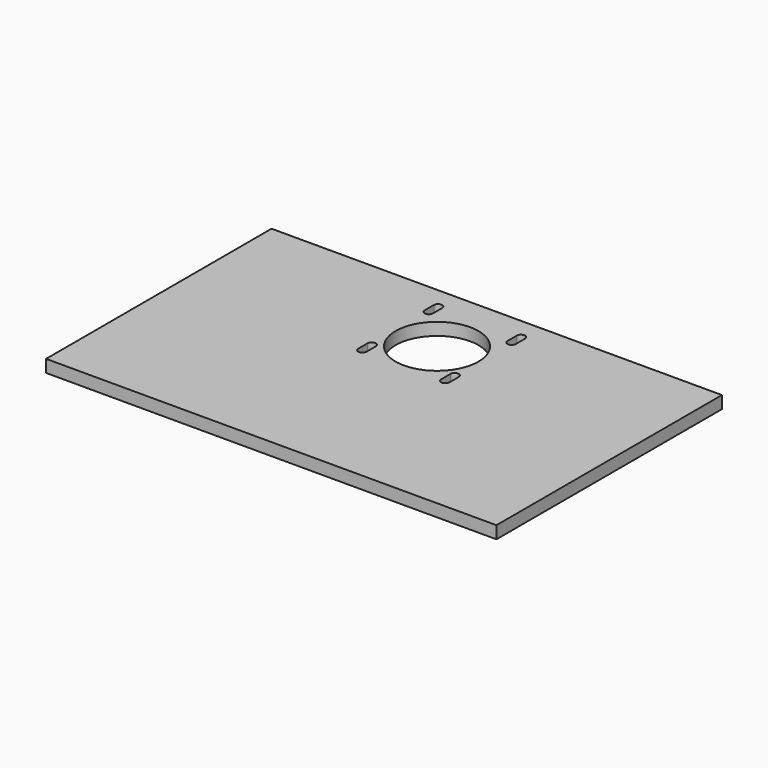
from build123d import *

# Parameters (mm, degrees)
F0_W     = 344.9914
F0_H     = 215.9
F0_R     = 31.75
F1_DEPTH = 9.525


# Not quite as in the source:
# - a length typed as a fraction of an inch, garbled in the dataset ("3 / 203.2 mm" for 3/8 in), is restored


with BuildPart() as f1:
    # F0 (on Top) → F1 (new body)
    with BuildSketch(Plane.XY):
        with Locations((0.0043, -50.8)):
            Rectangle(F0_W, F0_H)
        with BuildLine():
            ThreePointArc((-34.9247077073, -22.903081011), (-31.7715410013, -19.685073074), (-28.575, -22.86))
            Line((-28.575, -22.86), (-28.575, -31.75))
            ThreePointArc((-28.575, -31.75), (-31.7500524496, -34.9249999996), (-34.9249999983, -31.7498951008))
            Line((-34.9249999983, -31.7498951008), (-34.9247077073, -22.903081011))
        make_face(mode=Mode.SUBTRACT)
        Circle(F0_R, mode=Mode.SUBTRACT)
        with BuildLine():
            Line((-28.575, 40.64), (-28.575, 31.75))
            ThreePointArc((-28.575, 31.75), (-31.7500524496, 28.5750000004), (-34.9249999983, 31.7501048992))
            Line((-34.9249999983, 31.7501048992), (-34.9247077073, 40.596918989))
            ThreePointArc((-34.9247077073, 40.596918989), (-31.7715410013, 43.814926926), (-28.575, 40.64))
        make_face(mode=Mode.SUBTRACT)
        with BuildLine():
            ThreePointArc((28.5752922927, -22.903081011), (31.7284589987, -19.685073074), (34.925, -22.86))
            Line((34.925, -22.86), (34.925, -31.75))
            ThreePointArc((34.925, -31.75), (31.7499475504, -34.9249999996), (28.5750000017, -31.7498951008))
            Line((28.5750000017, -31.7498951008), (28.5752922927, -22.903081011))
        make_face(mode=Mode.SUBTRACT)
        with BuildLine():
            ThreePointArc((28.5752922927, 40.596918989), (31.7284589987, 43.814926926), (34.925, 40.64))
            Line((34.925, 40.64), (34.925, 31.75))
            ThreePointArc((34.925, 31.75), (31.7499475504, 28.5750000004), (28.5750000017, 31.7501048992))
            Line((28.5750000017, 31.7501048992), (28.5752922927, 40.596918989))
        make_face(mode=Mode.SUBTRACT)
    extrude(amount=F1_DEPTH)


solid = f1.part
